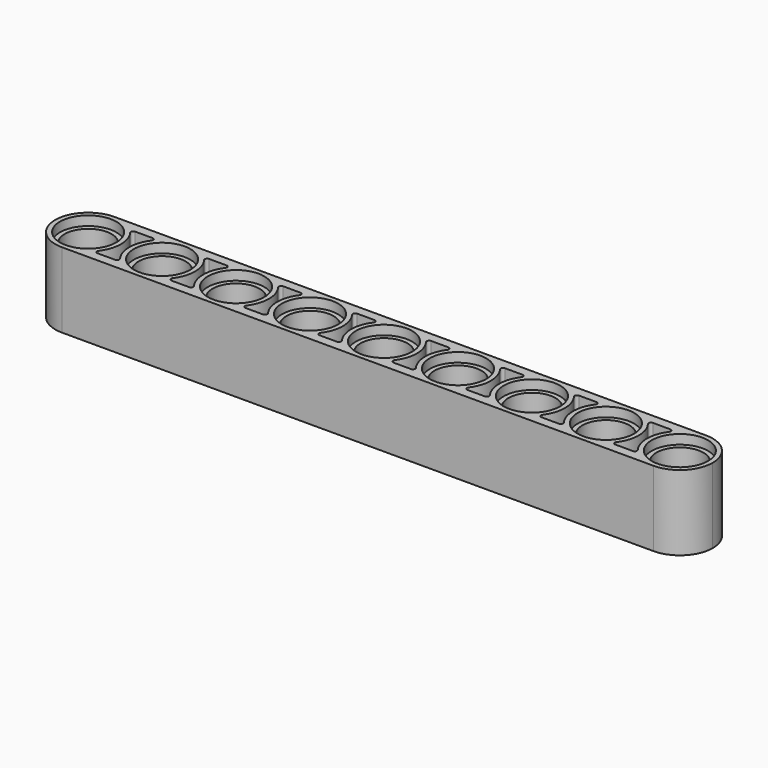
from build123d import *

# Parameters (mm, degrees)
F1_DEPTH  = 8
F2_R      = 2.5
F3_DEPTH  = 25
F2_R_2    = 3
F4_DEPTH  = 1
F5_R      = 3
F5_R_2    = 2.5
F6_DEPTH  = 1
F8_DEPTH  = 8
F9_DEPTH  = 4
F10_DEPTH = 3


# Not quite as in the source:
# - a feature names something its author has since deleted; it is built from what else it names


with BuildPart() as f1:
    # F0 (on Top) → F1 (new body)
    with BuildSketch(Plane.XY):
        with BuildLine():
            ThreePointArc((-40.6730920076, -45.3225079775), (-38.1982182735, -44.2973817116), (-37.1730920076, -41.8225079775))
            ThreePointArc((-37.1730920076, -41.8225079775), (-38.1982182735, -39.3476342433), (-40.6730920076, -38.3225079775))
            ThreePointArc((-40.6730920076, -38.3225079775), (-44.1730920076, -41.8225079775), (-40.6730920076, -45.3225079775))
        make_face()
        with BuildLine():
            Line((18.8269079924, -41.8225079775), (-37.1730920076, -41.8225079775))
            ThreePointArc((-37.1730920076, -41.8225079775), (-38.1982182735, -44.2973817116), (-40.6730920076, -45.3225079775))
            Line((-40.6730920076, -45.3225079775), (22.3269079924, -45.3225079775))
            ThreePointArc((22.3269079924, -45.3225079775), (19.8520342582, -44.2973817116), (18.8269079924, -41.8225079775))
        make_face()
        with BuildLine():
            ThreePointArc((-40.6730920076, -38.3225079775), (-38.1982182735, -39.3476342433), (-37.1730920076, -41.8225079775))
            Line((-37.1730920076, -41.8225079775), (18.8269079924, -41.8225079775))
            ThreePointArc((18.8269079924, -41.8225079775), (19.8520342582, -39.3476342433), (22.3269079924, -38.3225079775))
            Line((22.3269079924, -38.3225079775), (-40.6730920076, -38.3225079775))
        make_face()
        with BuildLine():
            ThreePointArc((22.3269079924, -38.3225079775), (19.8520342582, -39.3476342433), (18.8269079924, -41.8225079775))
            ThreePointArc((18.8269079924, -41.8225079775), (19.8520342582, -44.2973817116), (22.3269079924, -45.3225079775))
            ThreePointArc((22.3269079924, -45.3225079775), (24.8017817265, -44.2973817116), (25.8269079924, -41.8225079775))
            ThreePointArc((25.8269079924, -41.8225079775), (24.8017817265, -39.3476342433), (22.3269079924, -38.3225079775))
        make_face()
    extrude(amount=F1_DEPTH)

    # F2 (on face) → F3 (cut)
    with BuildSketch(Plane(origin=(0, 0, 0), x_dir=(1, 0, 0), z_dir=(0, 0, -1))):
        with Locations((-40.6730920076, 41.8225079775)):
            Circle(F2_R)
        with Locations((-32.7980920076, 41.8225079775)):
            Circle(F2_R)
        with Locations((-24.9230920076, 41.8225079775)):
            Circle(F2_R)
        with Locations((-17.0480920076, 41.8225079775)):
            Circle(F2_R)
        with Locations((-9.1730920076, 41.8225079775)):
            Circle(F2_R)
        with Locations((-1.2980920076, 41.8225079775)):
            Circle(F2_R)
        with Locations((6.5769079924, 41.8225079775)):
            Circle(F2_R)
        with Locations((14.4519079924, 41.8225079775)):
            Circle(F2_R)
        with Locations((22.3269079924, 41.8225079775)):
            Circle(F2_R)
    extrude(amount=-F3_DEPTH, mode=Mode.SUBTRACT)

    # F2 (on face) → F4 (cut)
    with BuildSketch(Plane(origin=(0, 0, 0), x_dir=(1, 0, 0), z_dir=(0, 0, -1))):
        with Locations((-40.6730920076, 41.8225079775)):
            Circle(F2_R_2)
        with Locations((-40.6730920076, 41.8225079775)):
            Circle(F2_R, mode=Mode.SUBTRACT)
        with Locations((-32.7980920076, 41.8225079775)):
            Circle(F2_R_2)
        with Locations((-32.7980920076, 41.8225079775)):
            Circle(F2_R, mode=Mode.SUBTRACT)
        with Locations((-24.9230920076, 41.8225079775)):
            Circle(F2_R_2)
        with Locations((-24.9230920076, 41.8225079775)):
            Circle(F2_R, mode=Mode.SUBTRACT)
        with Locations((-17.0480920076, 41.8225079775)):
            Circle(F2_R_2)
        with Locations((-17.0480920076, 41.8225079775)):
            Circle(F2_R, mode=Mode.SUBTRACT)
        with Locations((-9.1730920076, 41.8225079775)):
            Circle(F2_R_2)
        with Locations((-9.1730920076, 41.8225079775)):
            Circle(F2_R, mode=Mode.SUBTRACT)
        with Locations((-1.2980920076, 41.8225079775)):
            Circle(F2_R_2)
        with Locations((-1.2980920076, 41.8225079775)):
            Circle(F2_R, mode=Mode.SUBTRACT)
        with Locations((6.5769079924, 41.8225079775)):
            Circle(F2_R_2)
        with Locations((6.5769079924, 41.8225079775)):
            Circle(F2_R, mode=Mode.SUBTRACT)
        with Locations((14.4519079924, 41.8225079775)):
            Circle(F2_R_2)
        with Locations((14.4519079924, 41.8225079775)):
            Circle(F2_R, mode=Mode.SUBTRACT)
        with Locations((22.3269079924, 41.8225079775)):
            Circle(F2_R_2)
        with Locations((22.3269079924, 41.8225079775)):
            Circle(F2_R, mode=Mode.SUBTRACT)
    extrude(amount=-F4_DEPTH, mode=Mode.SUBTRACT)

    # F5 (on face) → F6 (cut)
    with BuildSketch(Plane.XY.offset(8)):
        with Locations((22.3269079924, -41.8225079775)):
            Circle(F5_R)
        with Locations((22.3269079924, -41.8225079775)):
            Circle(F5_R_2, mode=Mode.SUBTRACT)
        with Locations((14.4519079924, -41.8225079775)):
            Circle(F5_R)
        with Locations((14.4519079924, -41.8225079775)):
            Circle(F5_R_2, mode=Mode.SUBTRACT)
        with Locations((6.5769079924, -41.8225079775)):
            Circle(F5_R)
        with Locations((6.5769079924, -41.8225079775)):
            Circle(F5_R_2, mode=Mode.SUBTRACT)
        with Locations((-1.2980920076, -41.8225079775)):
            Circle(F5_R)
        with Locations((-1.2980920076, -41.8225079775)):
            Circle(F5_R_2, mode=Mode.SUBTRACT)
        with Locations((-9.1730920076, -41.8225079775)):
            Circle(F5_R)
        with Locations((-9.1730920076, -41.8225079775)):
            Circle(F5_R_2, mode=Mode.SUBTRACT)
        with Locations((-17.0480920076, -41.8225079775)):
            Circle(F5_R)
        with Locations((-17.0480920076, -41.8225079775)):
            Circle(F5_R_2, mode=Mode.SUBTRACT)
        with Locations((-24.9230920076, -41.8225079775)):
            Circle(F5_R)
        with Locations((-24.9230920076, -41.8225079775)):
            Circle(F5_R_2, mode=Mode.SUBTRACT)
        with Locations((-32.7980920076, -41.8225079775)):
            Circle(F5_R)
        with Locations((-32.7980920076, -41.8225079775)):
            Circle(F5_R_2, mode=Mode.SUBTRACT)
        with Locations((-40.6730920076, -41.8225079775)):
            Circle(F5_R)
        with Locations((-40.6730920076, -41.8225079775)):
            Circle(F5_R_2, mode=Mode.SUBTRACT)
    extrude(amount=-F6_DEPTH, mode=Mode.SUBTRACT)

    # F7 (on face) → F8 (cut)
    with BuildSketch(Plane.XY.offset(8)):
        with BuildLine():
            ThreePointArc((19.5239505298, -43.9185588984), (18.8269079924, -41.8225079775), (19.5239505298, -39.7264570565))
            ThreePointArc((19.5239505298, -39.7264570565), (19.5475140389, -39.4620081959), (19.3216199754, -39.3225079775))
            Line((19.3216199754, -39.3225079775), (17.4571960094, -39.3225079775))
            ThreePointArc((17.4571960094, -39.3225079775), (17.2313019458, -39.4620081959), (17.2548654549, -39.7264570565))
            ThreePointArc((17.2548654549, -39.7264570565), (17.9519079924, -41.8225079775), (17.2548654549, -43.9185588984))
            ThreePointArc((17.2548654549, -43.9185588984), (17.2313019458, -44.1830077591), (17.4571960094, -44.3225079775))
            Line((17.4571960094, -44.3225079775), (19.3216199754, -44.3225079775))
            ThreePointArc((19.3216199754, -44.3225079775), (19.5475140389, -44.1830077591), (19.5239505298, -43.9185588984))
        make_face()
        with BuildLine():
            ThreePointArc((11.6489505298, -43.9185588984), (10.9519079924, -41.8225079775), (11.6489505298, -39.7264570565))
            ThreePointArc((11.6489505298, -39.7264570565), (11.6725140389, -39.4620081959), (11.4466199754, -39.3225079775))
            Line((11.4466199754, -39.3225079775), (9.5821960094, -39.3225079775))
            ThreePointArc((9.5821960094, -39.3225079775), (9.3563019458, -39.4620081959), (9.3798654549, -39.7264570565))
            ThreePointArc((9.3798654549, -39.7264570565), (10.0769079924, -41.8225079775), (9.3798654549, -43.9185588984))
            ThreePointArc((9.3798654549, -43.9185588984), (9.3563019458, -44.1830077591), (9.5821960094, -44.3225079775))
            Line((9.5821960094, -44.3225079775), (11.4466199754, -44.3225079775))
            ThreePointArc((11.4466199754, -44.3225079775), (11.6725140389, -44.1830077591), (11.6489505298, -43.9185588984))
        make_face()
        with BuildLine():
            ThreePointArc((3.7739505298, -43.9185588984), (3.0769079924, -41.8225079775), (3.7739505298, -39.7264570565))
            ThreePointArc((3.7739505298, -39.7264570565), (3.7975140389, -39.4620081959), (3.5716199754, -39.3225079775))
            Line((3.5716199754, -39.3225079775), (1.7071960094, -39.3225079775))
            ThreePointArc((1.7071960094, -39.3225079775), (1.4813019458, -39.4620081959), (1.5048654549, -39.7264570565))
            ThreePointArc((1.5048654549, -39.7264570565), (2.2019079924, -41.8225079775), (1.5048654549, -43.9185588984))
            ThreePointArc((1.5048654549, -43.9185588984), (1.4813019458, -44.1830077591), (1.7071960094, -44.3225079775))
            Line((1.7071960094, -44.3225079775), (3.5716199754, -44.3225079775))
            ThreePointArc((3.5716199754, -44.3225079775), (3.7975140389, -44.1830077591), (3.7739505298, -43.9185588984))
        make_face()
        with BuildLine():
            ThreePointArc((-4.1010494702, -43.9185588984), (-4.7980920076, -41.8225079775), (-4.1010494702, -39.7264570565))
            ThreePointArc((-4.1010494702, -39.7264570565), (-4.0774859611, -39.4620081959), (-4.3033800246, -39.3225079775))
            Line((-4.3033800246, -39.3225079775), (-6.1678039906, -39.3225079775))
            ThreePointArc((-6.1678039906, -39.3225079775), (-6.3936980542, -39.4620081959), (-6.3701345451, -39.7264570565))
            ThreePointArc((-6.3701345451, -39.7264570565), (-5.6730920076, -41.8225079775), (-6.3701345451, -43.9185588984))
            ThreePointArc((-6.3701345451, -43.9185588984), (-6.3936980542, -44.1830077591), (-6.1678039906, -44.3225079775))
            Line((-6.1678039906, -44.3225079775), (-4.3033800246, -44.3225079775))
            ThreePointArc((-4.3033800246, -44.3225079775), (-4.0774859611, -44.1830077591), (-4.1010494702, -43.9185588984))
        make_face()
        with BuildLine():
            ThreePointArc((-11.9760494702, -43.9185588984), (-12.6730920076, -41.8225079775), (-11.9760494702, -39.7264570565))
            ThreePointArc((-11.9760494702, -39.7264570565), (-11.9524859611, -39.4620081959), (-12.1783800246, -39.3225079775))
            Line((-12.1783800246, -39.3225079775), (-14.0428039906, -39.3225079775))
            ThreePointArc((-14.0428039906, -39.3225079775), (-14.2686980542, -39.4620081959), (-14.2451345451, -39.7264570565))
            ThreePointArc((-14.2451345451, -39.7264570565), (-13.5480920076, -41.8225079775), (-14.2451345451, -43.9185588984))
            ThreePointArc((-14.2451345451, -43.9185588984), (-14.2686980542, -44.1830077591), (-14.0428039906, -44.3225079775))
            Line((-14.0428039906, -44.3225079775), (-12.1783800246, -44.3225079775))
            ThreePointArc((-12.1783800246, -44.3225079775), (-11.9524859611, -44.1830077591), (-11.9760494702, -43.9185588984))
        make_face()
        with BuildLine():
            ThreePointArc((-19.8510494702, -43.9185588984), (-20.5480920076, -41.8225079775), (-19.8510494702, -39.7264570565))
            ThreePointArc((-19.8510494702, -39.7264570565), (-19.8274859611, -39.4620081959), (-20.0533800246, -39.3225079775))
            Line((-20.0533800246, -39.3225079775), (-21.9178039906, -39.3225079775))
            ThreePointArc((-21.9178039906, -39.3225079775), (-22.1436980542, -39.4620081959), (-22.1201345451, -39.7264570565))
            ThreePointArc((-22.1201345451, -39.7264570565), (-21.4230920076, -41.8225079775), (-22.1201345451, -43.9185588984))
            ThreePointArc((-22.1201345451, -43.9185588984), (-22.1436980542, -44.1830077591), (-21.9178039906, -44.3225079775))
            Line((-21.9178039906, -44.3225079775), (-20.0533800246, -44.3225079775))
            ThreePointArc((-20.0533800246, -44.3225079775), (-19.8274859611, -44.1830077591), (-19.8510494702, -43.9185588984))
        make_face()
        with BuildLine():
            ThreePointArc((-35.6010494702, -43.9185588984), (-36.2980920076, -41.8225079775), (-35.6010494702, -39.7264570565))
            ThreePointArc((-35.6010494702, -39.7264570565), (-35.5774859611, -39.4620081959), (-35.8033800246, -39.3225079775))
            Line((-35.8033800246, -39.3225079775), (-37.6678039906, -39.3225079775))
            ThreePointArc((-37.6678039906, -39.3225079775), (-37.8936980542, -39.4620081959), (-37.8701345451, -39.7264570565))
            ThreePointArc((-37.8701345451, -39.7264570565), (-37.1730920076, -41.8225079775), (-37.8701345451, -43.9185588984))
            ThreePointArc((-37.8701345451, -43.9185588984), (-37.8936980542, -44.1830077591), (-37.6678039906, -44.3225079775))
            Line((-37.6678039906, -44.3225079775), (-35.8033800246, -44.3225079775))
            ThreePointArc((-35.8033800246, -44.3225079775), (-35.5774859611, -44.1830077591), (-35.6010494702, -43.9185588984))
        make_face()
        with BuildLine():
            ThreePointArc((-27.7260494702, -43.9185588984), (-28.4230920076, -41.8225079775), (-27.7260494702, -39.7264570565))
            ThreePointArc((-27.7260494702, -39.7264570565), (-27.7024859611, -39.4620081959), (-27.9283800246, -39.3225079775))
            Line((-27.9283800246, -39.3225079775), (-29.7928039906, -39.3225079775))
            ThreePointArc((-29.7928039906, -39.3225079775), (-30.0186980542, -39.4620081959), (-29.9951345451, -39.7264570565))
            ThreePointArc((-29.9951345451, -39.7264570565), (-29.2980920076, -41.8225079775), (-29.9951345451, -43.9185588984))
            ThreePointArc((-29.9951345451, -43.9185588984), (-30.0186980542, -44.1830077591), (-29.7928039906, -44.3225079775))
            Line((-29.7928039906, -44.3225079775), (-27.9283800246, -44.3225079775))
            ThreePointArc((-27.9283800246, -44.3225079775), (-27.7024859611, -44.1830077591), (-27.7260494702, -43.9185588984))
        make_face()
    extrude(amount=-F8_DEPTH, mode=Mode.SUBTRACT)

    # F7 (on face) → F9 (join)
    with BuildSketch(Plane.XY.offset(8)):
        with BuildLine():
            ThreePointArc((19.5239505298, -43.9185588984), (18.8269079924, -41.8225079775), (19.5239505298, -39.7264570565))
            ThreePointArc((19.5239505298, -39.7264570565), (19.5475140389, -39.4620081959), (19.3216199754, -39.3225079775))
            Line((19.3216199754, -39.3225079775), (17.4571960094, -39.3225079775))
            ThreePointArc((17.4571960094, -39.3225079775), (17.2313019458, -39.4620081959), (17.2548654549, -39.7264570565))
            ThreePointArc((17.2548654549, -39.7264570565), (17.9519079924, -41.8225079775), (17.2548654549, -43.9185588984))
            ThreePointArc((17.2548654549, -43.9185588984), (17.2313019458, -44.1830077591), (17.4571960094, -44.3225079775))
            Line((17.4571960094, -44.3225079775), (19.3216199754, -44.3225079775))
            ThreePointArc((19.3216199754, -44.3225079775), (19.5475140389, -44.1830077591), (19.5239505298, -43.9185588984))
        make_face()
        with BuildLine():
            ThreePointArc((11.6489505298, -43.9185588984), (10.9519079924, -41.8225079775), (11.6489505298, -39.7264570565))
            ThreePointArc((11.6489505298, -39.7264570565), (11.6725140389, -39.4620081959), (11.4466199754, -39.3225079775))
            Line((11.4466199754, -39.3225079775), (9.5821960094, -39.3225079775))
            ThreePointArc((9.5821960094, -39.3225079775), (9.3563019458, -39.4620081959), (9.3798654549, -39.7264570565))
            ThreePointArc((9.3798654549, -39.7264570565), (10.0769079924, -41.8225079775), (9.3798654549, -43.9185588984))
            ThreePointArc((9.3798654549, -43.9185588984), (9.3563019458, -44.1830077591), (9.5821960094, -44.3225079775))
            Line((9.5821960094, -44.3225079775), (11.4466199754, -44.3225079775))
            ThreePointArc((11.4466199754, -44.3225079775), (11.6725140389, -44.1830077591), (11.6489505298, -43.9185588984))
        make_face()
        with BuildLine():
            ThreePointArc((3.7739505298, -43.9185588984), (3.0769079924, -41.8225079775), (3.7739505298, -39.7264570565))
            ThreePointArc((3.7739505298, -39.7264570565), (3.7975140389, -39.4620081959), (3.5716199754, -39.3225079775))
            Line((3.5716199754, -39.3225079775), (1.7071960094, -39.3225079775))
            ThreePointArc((1.7071960094, -39.3225079775), (1.4813019458, -39.4620081959), (1.5048654549, -39.7264570565))
            ThreePointArc((1.5048654549, -39.7264570565), (2.2019079924, -41.8225079775), (1.5048654549, -43.9185588984))
            ThreePointArc((1.5048654549, -43.9185588984), (1.4813019458, -44.1830077591), (1.7071960094, -44.3225079775))
            Line((1.7071960094, -44.3225079775), (3.5716199754, -44.3225079775))
            ThreePointArc((3.5716199754, -44.3225079775), (3.7975140389, -44.1830077591), (3.7739505298, -43.9185588984))
        make_face()
        with BuildLine():
            ThreePointArc((-4.1010494702, -43.9185588984), (-4.7980920076, -41.8225079775), (-4.1010494702, -39.7264570565))
            ThreePointArc((-4.1010494702, -39.7264570565), (-4.0774859611, -39.4620081959), (-4.3033800246, -39.3225079775))
            Line((-4.3033800246, -39.3225079775), (-6.1678039906, -39.3225079775))
            ThreePointArc((-6.1678039906, -39.3225079775), (-6.3936980542, -39.4620081959), (-6.3701345451, -39.7264570565))
            ThreePointArc((-6.3701345451, -39.7264570565), (-5.6730920076, -41.8225079775), (-6.3701345451, -43.9185588984))
            ThreePointArc((-6.3701345451, -43.9185588984), (-6.3936980542, -44.1830077591), (-6.1678039906, -44.3225079775))
            Line((-6.1678039906, -44.3225079775), (-4.3033800246, -44.3225079775))
            ThreePointArc((-4.3033800246, -44.3225079775), (-4.0774859611, -44.1830077591), (-4.1010494702, -43.9185588984))
        make_face()
        with BuildLine():
            ThreePointArc((-11.9760494702, -43.9185588984), (-12.6730920076, -41.8225079775), (-11.9760494702, -39.7264570565))
            ThreePointArc((-11.9760494702, -39.7264570565), (-11.9524859611, -39.4620081959), (-12.1783800246, -39.3225079775))
            Line((-12.1783800246, -39.3225079775), (-14.0428039906, -39.3225079775))
            ThreePointArc((-14.0428039906, -39.3225079775), (-14.2686980542, -39.4620081959), (-14.2451345451, -39.7264570565))
            ThreePointArc((-14.2451345451, -39.7264570565), (-13.5480920076, -41.8225079775), (-14.2451345451, -43.9185588984))
            ThreePointArc((-14.2451345451, -43.9185588984), (-14.2686980542, -44.1830077591), (-14.0428039906, -44.3225079775))
            Line((-14.0428039906, -44.3225079775), (-12.1783800246, -44.3225079775))
            ThreePointArc((-12.1783800246, -44.3225079775), (-11.9524859611, -44.1830077591), (-11.9760494702, -43.9185588984))
        make_face()
        with BuildLine():
            ThreePointArc((-19.8510494702, -43.9185588984), (-20.5480920076, -41.8225079775), (-19.8510494702, -39.7264570565))
            ThreePointArc((-19.8510494702, -39.7264570565), (-19.8274859611, -39.4620081959), (-20.0533800246, -39.3225079775))
            Line((-20.0533800246, -39.3225079775), (-21.9178039906, -39.3225079775))
            ThreePointArc((-21.9178039906, -39.3225079775), (-22.1436980542, -39.4620081959), (-22.1201345451, -39.7264570565))
            ThreePointArc((-22.1201345451, -39.7264570565), (-21.4230920076, -41.8225079775), (-22.1201345451, -43.9185588984))
            ThreePointArc((-22.1201345451, -43.9185588984), (-22.1436980542, -44.1830077591), (-21.9178039906, -44.3225079775))
            Line((-21.9178039906, -44.3225079775), (-20.0533800246, -44.3225079775))
            ThreePointArc((-20.0533800246, -44.3225079775), (-19.8274859611, -44.1830077591), (-19.8510494702, -43.9185588984))
        make_face()
        with BuildLine():
            ThreePointArc((-27.7260494702, -43.9185588984), (-28.4230920076, -41.8225079775), (-27.7260494702, -39.7264570565))
            ThreePointArc((-27.7260494702, -39.7264570565), (-27.7024859611, -39.4620081959), (-27.9283800246, -39.3225079775))
            Line((-27.9283800246, -39.3225079775), (-29.7928039906, -39.3225079775))
            ThreePointArc((-29.7928039906, -39.3225079775), (-30.0186980542, -39.4620081959), (-29.9951345451, -39.7264570565))
            ThreePointArc((-29.9951345451, -39.7264570565), (-29.2980920076, -41.8225079775), (-29.9951345451, -43.9185588984))
            ThreePointArc((-29.9951345451, -43.9185588984), (-30.0186980542, -44.1830077591), (-29.7928039906, -44.3225079775))
            Line((-29.7928039906, -44.3225079775), (-27.9283800246, -44.3225079775))
            ThreePointArc((-27.9283800246, -44.3225079775), (-27.7024859611, -44.1830077591), (-27.7260494702, -43.9185588984))
        make_face()
        with BuildLine():
            ThreePointArc((-35.6010494702, -43.9185588984), (-36.2980920076, -41.8225079775), (-35.6010494702, -39.7264570565))
            ThreePointArc((-35.6010494702, -39.7264570565), (-35.5774859611, -39.4620081959), (-35.8033800246, -39.3225079775))
            Line((-35.8033800246, -39.3225079775), (-37.6678039906, -39.3225079775))
            ThreePointArc((-37.6678039906, -39.3225079775), (-37.8936980542, -39.4620081959), (-37.8701345451, -39.7264570565))
            ThreePointArc((-37.8701345451, -39.7264570565), (-37.1730920076, -41.8225079775), (-37.8701345451, -43.9185588984))
            ThreePointArc((-37.8701345451, -43.9185588984), (-37.8936980542, -44.1830077591), (-37.6678039906, -44.3225079775))
            Line((-37.6678039906, -44.3225079775), (-35.8033800246, -44.3225079775))
            ThreePointArc((-35.8033800246, -44.3225079775), (-35.5774859611, -44.1830077591), (-35.6010494702, -43.9185588984))
        make_face()
    extrude(amount=-F9_DEPTH)

    # F7 (on face) → F10 (cut)
    with BuildSketch(Plane.XY.offset(8)):
        with BuildLine():
            ThreePointArc((19.5239505298, -43.9185588984), (18.8269079924, -41.8225079775), (19.5239505298, -39.7264570565))
            ThreePointArc((19.5239505298, -39.7264570565), (19.5475140389, -39.4620081959), (19.3216199754, -39.3225079775))
            Line((19.3216199754, -39.3225079775), (17.4571960094, -39.3225079775))
            ThreePointArc((17.4571960094, -39.3225079775), (17.2313019458, -39.4620081959), (17.2548654549, -39.7264570565))
            ThreePointArc((17.2548654549, -39.7264570565), (17.9519079924, -41.8225079775), (17.2548654549, -43.9185588984))
            ThreePointArc((17.2548654549, -43.9185588984), (17.2313019458, -44.1830077591), (17.4571960094, -44.3225079775))
            Line((17.4571960094, -44.3225079775), (19.3216199754, -44.3225079775))
            ThreePointArc((19.3216199754, -44.3225079775), (19.5475140389, -44.1830077591), (19.5239505298, -43.9185588984))
        make_face()
        with BuildLine():
            ThreePointArc((11.6489505298, -43.9185588984), (10.9519079924, -41.8225079775), (11.6489505298, -39.7264570565))
            ThreePointArc((11.6489505298, -39.7264570565), (11.6725140389, -39.4620081959), (11.4466199754, -39.3225079775))
            Line((11.4466199754, -39.3225079775), (9.5821960094, -39.3225079775))
            ThreePointArc((9.5821960094, -39.3225079775), (9.3563019458, -39.4620081959), (9.3798654549, -39.7264570565))
            ThreePointArc((9.3798654549, -39.7264570565), (10.0769079924, -41.8225079775), (9.3798654549, -43.9185588984))
            ThreePointArc((9.3798654549, -43.9185588984), (9.3563019458, -44.1830077591), (9.5821960094, -44.3225079775))
            Line((9.5821960094, -44.3225079775), (11.4466199754, -44.3225079775))
            ThreePointArc((11.4466199754, -44.3225079775), (11.6725140389, -44.1830077591), (11.6489505298, -43.9185588984))
        make_face()
        with BuildLine():
            ThreePointArc((3.7739505298, -43.9185588984), (3.0769079924, -41.8225079775), (3.7739505298, -39.7264570565))
            ThreePointArc((3.7739505298, -39.7264570565), (3.7975140389, -39.4620081959), (3.5716199754, -39.3225079775))
            Line((3.5716199754, -39.3225079775), (1.7071960094, -39.3225079775))
            ThreePointArc((1.7071960094, -39.3225079775), (1.4813019458, -39.4620081959), (1.5048654549, -39.7264570565))
            ThreePointArc((1.5048654549, -39.7264570565), (2.2019079924, -41.8225079775), (1.5048654549, -43.9185588984))
            ThreePointArc((1.5048654549, -43.9185588984), (1.4813019458, -44.1830077591), (1.7071960094, -44.3225079775))
            Line((1.7071960094, -44.3225079775), (3.5716199754, -44.3225079775))
            ThreePointArc((3.5716199754, -44.3225079775), (3.7975140389, -44.1830077591), (3.7739505298, -43.9185588984))
        make_face()
        with BuildLine():
            ThreePointArc((-4.1010494702, -43.9185588984), (-4.7980920076, -41.8225079775), (-4.1010494702, -39.7264570565))
            ThreePointArc((-4.1010494702, -39.7264570565), (-4.0774859611, -39.4620081959), (-4.3033800246, -39.3225079775))
            Line((-4.3033800246, -39.3225079775), (-6.1678039906, -39.3225079775))
            ThreePointArc((-6.1678039906, -39.3225079775), (-6.3936980542, -39.4620081959), (-6.3701345451, -39.7264570565))
            ThreePointArc((-6.3701345451, -39.7264570565), (-5.6730920076, -41.8225079775), (-6.3701345451, -43.9185588984))
            ThreePointArc((-6.3701345451, -43.9185588984), (-6.3936980542, -44.1830077591), (-6.1678039906, -44.3225079775))
            Line((-6.1678039906, -44.3225079775), (-4.3033800246, -44.3225079775))
            ThreePointArc((-4.3033800246, -44.3225079775), (-4.0774859611, -44.1830077591), (-4.1010494702, -43.9185588984))
        make_face()
        with BuildLine():
            ThreePointArc((-11.9760494702, -43.9185588984), (-12.6730920076, -41.8225079775), (-11.9760494702, -39.7264570565))
            ThreePointArc((-11.9760494702, -39.7264570565), (-11.9524859611, -39.4620081959), (-12.1783800246, -39.3225079775))
            Line((-12.1783800246, -39.3225079775), (-14.0428039906, -39.3225079775))
            ThreePointArc((-14.0428039906, -39.3225079775), (-14.2686980542, -39.4620081959), (-14.2451345451, -39.7264570565))
            ThreePointArc((-14.2451345451, -39.7264570565), (-13.5480920076, -41.8225079775), (-14.2451345451, -43.9185588984))
            ThreePointArc((-14.2451345451, -43.9185588984), (-14.2686980542, -44.1830077591), (-14.0428039906, -44.3225079775))
            Line((-14.0428039906, -44.3225079775), (-12.1783800246, -44.3225079775))
            ThreePointArc((-12.1783800246, -44.3225079775), (-11.9524859611, -44.1830077591), (-11.9760494702, -43.9185588984))
        make_face()
        with BuildLine():
            ThreePointArc((-19.8510494702, -43.9185588984), (-20.5480920076, -41.8225079775), (-19.8510494702, -39.7264570565))
            ThreePointArc((-19.8510494702, -39.7264570565), (-19.8274859611, -39.4620081959), (-20.0533800246, -39.3225079775))
            Line((-20.0533800246, -39.3225079775), (-21.9178039906, -39.3225079775))
            ThreePointArc((-21.9178039906, -39.3225079775), (-22.1436980542, -39.4620081959), (-22.1201345451, -39.7264570565))
            ThreePointArc((-22.1201345451, -39.7264570565), (-21.4230920076, -41.8225079775), (-22.1201345451, -43.9185588984))
            ThreePointArc((-22.1201345451, -43.9185588984), (-22.1436980542, -44.1830077591), (-21.9178039906, -44.3225079775))
            Line((-21.9178039906, -44.3225079775), (-20.0533800246, -44.3225079775))
            ThreePointArc((-20.0533800246, -44.3225079775), (-19.8274859611, -44.1830077591), (-19.8510494702, -43.9185588984))
        make_face()
        with BuildLine():
            ThreePointArc((-27.7260494702, -43.9185588984), (-28.4230920076, -41.8225079775), (-27.7260494702, -39.7264570565))
            ThreePointArc((-27.7260494702, -39.7264570565), (-27.7024859611, -39.4620081959), (-27.9283800246, -39.3225079775))
            Line((-27.9283800246, -39.3225079775), (-29.7928039906, -39.3225079775))
            ThreePointArc((-29.7928039906, -39.3225079775), (-30.0186980542, -39.4620081959), (-29.9951345451, -39.7264570565))
            ThreePointArc((-29.9951345451, -39.7264570565), (-29.2980920076, -41.8225079775), (-29.9951345451, -43.9185588984))
            ThreePointArc((-29.9951345451, -43.9185588984), (-30.0186980542, -44.1830077591), (-29.7928039906, -44.3225079775))
            Line((-29.7928039906, -44.3225079775), (-27.9283800246, -44.3225079775))
            ThreePointArc((-27.9283800246, -44.3225079775), (-27.7024859611, -44.1830077591), (-27.7260494702, -43.9185588984))
        make_face()
        with BuildLine():
            ThreePointArc((-35.6010494702, -43.9185588984), (-36.2980920076, -41.8225079775), (-35.6010494702, -39.7264570565))
            ThreePointArc((-35.6010494702, -39.7264570565), (-35.5774859611, -39.4620081959), (-35.8033800246, -39.3225079775))
            Line((-35.8033800246, -39.3225079775), (-37.6678039906, -39.3225079775))
            ThreePointArc((-37.6678039906, -39.3225079775), (-37.8936980542, -39.4620081959), (-37.8701345451, -39.7264570565))
            ThreePointArc((-37.8701345451, -39.7264570565), (-37.1730920076, -41.8225079775), (-37.8701345451, -43.9185588984))
            ThreePointArc((-37.8701345451, -43.9185588984), (-37.8936980542, -44.1830077591), (-37.6678039906, -44.3225079775))
            Line((-37.6678039906, -44.3225079775), (-35.8033800246, -44.3225079775))
            ThreePointArc((-35.8033800246, -44.3225079775), (-35.5774859611, -44.1830077591), (-35.6010494702, -43.9185588984))
        make_face()
    extrude(amount=-F10_DEPTH, mode=Mode.SUBTRACT)


solid = f1.part
